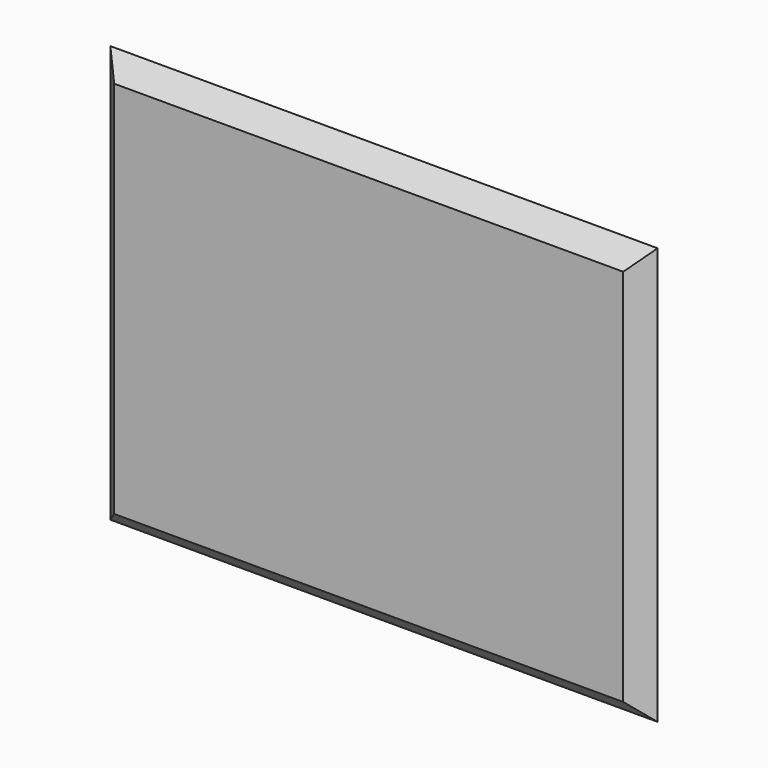
from build123d import *

# Parameters (mm, degrees)
F0_W     = 630
F0_H     = 480
F1_DEPTH = 22
F2_SIZE  = 21.99999


# Not quite as in the source:
# - a fillet or chamfer is up to 0.001 mm smaller than in the source, because OpenCascade refuses the exact size


with BuildPart() as f1:
    # F0 (on Front) → F1 (new body)
    with BuildSketch(Plane.XZ):
        Rectangle(F0_W, F0_H)
    extrude(amount=F1_DEPTH)

    # F2 (size 22 in the source; OpenCascade refuses exactly that, so slightly less here)
    f2_edges = [f1.edges().sort_by_distance(p)[0] for p in [
        (-315, -22, 0),
        (0, -22, 240),
        (315, -22, 0),
        (0, -22, -240),
    ]]
    chamfer(f2_edges, length=F2_SIZE)


solid = f1.part
